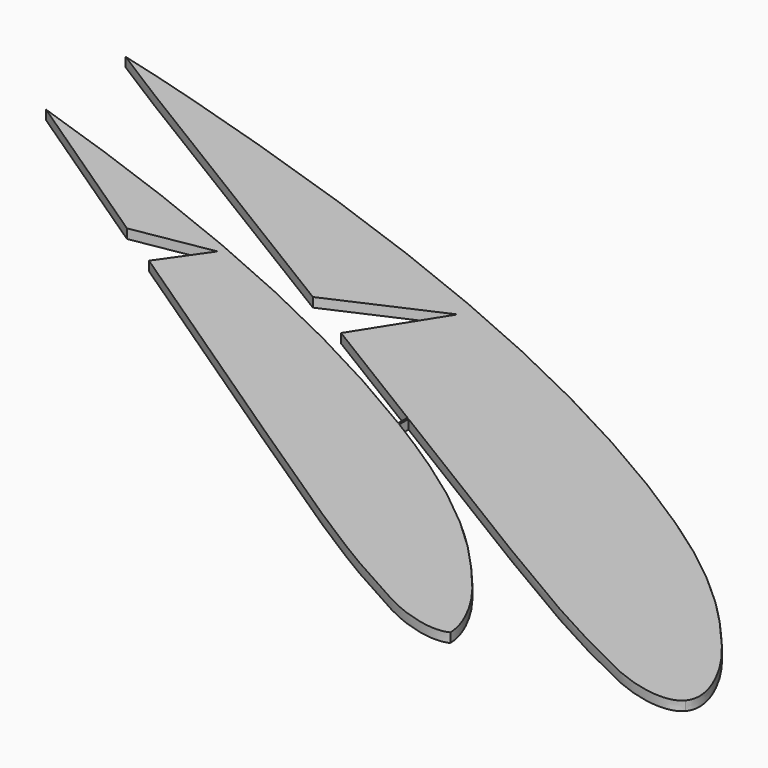
from build123d import *

# Parameters (mm, degrees)
F1_DEPTH = 2


# Not quite as in the source:
# - the dataset's text gives a spline's control points without its knots; the knots are read off the source's solid
# - a feature names something its author has since deleted; it is built from what else it names


with BuildPart() as f1:
    # F0 (on Top) → F1 (new body)
    with BuildSketch(Plane.XY):
        with BuildLine():
            add(Edge.make_bspline(
                [(34.860599786, 6.0687586182), (35.2687453157, 5.8190452704), (37.9503490475, 4.1782223052), (42.9046433804, 1.1446644855), (49.7245476866, -3.027837403), (56.54608151, -7.2008211399), (63.3647574685, -11.3765509779), (69.0485632229, -14.8494069376), (73.6045415108, -17.6232662722), (77.0228874716, -19.7002862098), (80.4388440403, -21.7712172731), (83.8571502757, -23.8323742426), (86.7081675393, -25.5302350613), (89.0084243125, -26.8828856902), (90.7408045712, -27.8935456128), (92.4769612198, -28.8998816401), (94.2144438156, -29.9024682228), (95.9476947005, -30.8994796567), (97.67369129, -31.889003941), (99.3967456723, -32.8707532075), (101.126358674, -33.8441717679), (102.8704996688, -34.8067332872), (104.6349485728, -35.7562751813), (106.4257836837, -36.6941374387), (108.2368428496, -37.6199323622), (110.0525217909, -38.5337763803), (111.8555610734, -39.4368456272), (113.6278147654, -40.3278884849), (115.3611971774, -41.2041212919), (117.0700429624, -42.0607550761), (118.7971750388, -42.8873919534), (120.2987360559, -43.539044525), (121.5536357842, -44.027474014), (122.8468885355, -44.4903446585), (124.531625858, -45.0115374905), (126.6377529307, -45.5104636967), (128.4270481511, -45.7764347039), (129.8441585723, -45.8545335174), (130.8873251545, -45.8291031583), (131.8926379099, -45.6988700343), (132.828483914, -45.43983661), (133.6579819463, -45.0271299968), (134.1089517191, -44.6391463008), (134.3025347026, -44.4182446105)],
                knots=[805.0679993481, 805.0679993481, 805.0679993481, 805.0679993481, 813.1781775179, 858.3547429355, 903.5313083532, 948.7078737709, 993.8844391885, 1039.0610046062, 1061.649287315, 1084.2375700238, 1106.8258527327, 1129.4141354415, 1152.0024181503, 1163.2965595047, 1174.5907008592, 1185.8848422136, 1197.178983568, 1208.4731249224, 1219.7672662768, 1231.0614076312, 1242.3555489857, 1253.6496903401, 1264.9438316945, 1276.2379730489, 1287.5321144033, 1298.8262557577, 1310.1203971121, 1321.4145384666, 1332.708679821, 1344.0028211754, 1355.2969625298, 1366.5911038842, 1372.2381745614, 1377.8852452386, 1389.179386593, 1400.4735279475, 1411.7676693019, 1417.4147399791, 1423.0618106563, 1428.7088813335, 1434.3559520107, 1440.0030226879, 1445.6500933651, 1445.6500933651, 1445.6500933651, 1445.6500933651], degree=3))
            add(Edge.make_bspline(
                [(134.3025347026, -44.4182446105), (134.4985490764, -44.1945684086), (134.8248159243, -43.6923009831), (135.1078544695, -42.8095001783), (135.205021821, -41.8422445125), (135.1501095293, -40.8282113605), (134.975391368, -39.7894708339), (134.7075732398, -38.7435385922), (134.3683354813, -37.7026123972), (133.841804506, -36.3291331372), (133.0760844187, -34.6508561389), (132.0561245272, -32.7309758173), (131.1567589387, -31.2285596568), (130.4187876834, -30.0885083492), (129.8574307231, -29.2631222798), (129.2885766755, -28.4642996802), (128.7105806023, -27.6857239166), (128.1224667089, -26.9217345108), (127.5240892916, -26.1675844071), (126.9126520377, -25.4155593408), (126.0792163914, -24.4101439472), (125.0044725273, -23.14313805), (123.6727030697, -21.6085195966), (122.3086179596, -20.0710503087), (120.9197072947, -18.544727339), (119.5127808585, -17.0448685527), (118.0906248287, -15.5804853344), (116.6556539097, -14.1561713196), (115.2043354173, -12.7670509391), (113.731067744, -11.4038507997), (112.2359474887, -10.06162161), (110.2113517993, -8.2930831737), (107.6229635156, -6.1178813566), (104.4430145695, -3.5839997225), (101.2076134278, -1.1457368322), (97.9237908915, 1.2091018409), (94.5952853786, 3.5053295316), (91.228268046, 5.7578295955), (86.7000179994, 8.7039617459), (82.1227805571, 11.5638270054), (77.5023902987, 14.3514293201), (74.0156610077, 16.4084086641), (70.5081197823, 18.4312591562), (66.983191083, 20.4179504986), (63.4382661844, 22.3714369923), (58.6877730154, 24.9332961185), (52.7131711017, 28.0551419964), (46.6806069198, 31.0762775575), (41.8235450338, 33.4337885791), (38.1655202683, 35.1733203209), (34.494587003, 36.8840687288), (29.5847481148, 39.1269405961), (23.4177587851, 41.8613078428), (17.2165224292, 44.5057919901), (12.2323115482, 46.572058939), (8.4826600104, 48.0979477813), (4.7239527171, 49.5999016999), (-0.2907115865, 51.5680807839), (-6.5621137407, 53.9644562837), (-12.864106821, 56.2905039474), (-17.9365378549, 58.1171933612), (-21.7532419819, 59.4699275213), (-25.5722099127, 60.8026890188), (-29.3902027457, 62.1148948136), (-33.2135123019, 63.4090298901), (-36.4095997856, 64.4746966143), (-38.972432745, 65.3199824625), (-41.537052636, 66.1599255834), (-46.0356987638, 67.6183180092), (-50.5544663128, 69.0533041025), (-54.4226479189, 70.2589031341), (-56.3562208186, 70.857081615), (-58.2915278, 71.4515221165), (-60.2400882209, 72.0459223863), (-62.1998296313, 72.639688125), (-64.1623631317, 73.2301356662), (-66.1185814879, 73.8141454773), (-68.0631750531, 74.3895135617), (-70.0051537093, 74.9580604377), (-71.9471572764, 75.5195749662), (-73.8864183513, 76.0723784332), (-76.4709863037, 76.7976496792), (-79.7065256164, 77.6826704392), (-82.3144423774, 78.3701151223), (-83.6209282279, 78.7080004811)],
                knots=[0, 0, 0, 0, 5.7179975377, 11.4359950753, 17.153992613, 22.8719901506, 28.5899876883, 34.3079852259, 40.0259827636, 45.7439803013, 57.1799753766, 68.6159704519, 80.0519655272, 85.7699630649, 91.4879606025, 97.2059581402, 102.9239556778, 108.6419532155, 114.3599507531, 120.0779482908, 125.7959458284, 137.2319409038, 148.6679359791, 160.1039310544, 171.5399261297, 182.975921205, 194.4119162803, 205.8479113556, 217.283906431, 228.7199015063, 240.1558965816, 251.5918916569, 274.4638818075, 297.3358719582, 320.2078621088, 343.0798522594, 365.95184241, 388.8238325607, 411.6958227113, 457.4398030125, 480.3117931632, 503.1837833138, 526.0557734644, 548.927763615, 571.7997537657, 594.6717439163, 640.4157242176, 686.1597045188, 709.0316946694, 731.9036848201, 754.7756749707, 777.6476651213, 823.3916454226, 869.1356257238, 892.0076158745, 914.8796060251, 937.7515961757, 960.6235863263, 1006.3675666276, 1052.1115469288, 1074.9835370795, 1097.8555272301, 1120.7275173807, 1143.5995075313, 1166.471497682, 1189.3434878326, 1200.7794829079, 1212.2154779832, 1235.0874681339, 1280.8314484351, 1292.2674435104, 1303.7034385857, 1315.139433661, 1326.5754287364, 1338.0114238117, 1349.447418887, 1360.8834139623, 1372.3194090376, 1383.7554041129, 1395.1913991882, 1406.6273942636, 1418.0633893389, 1440.9353794895, 1463.8073696401, 1463.8073696401, 1463.8073696401, 1463.8073696401], degree=3))
            add(Edge.make_bspline(
                [(-83.6209282279, 78.7080004811), (-82.4998479043, 77.9874443746), (-80.2533908905, 76.553211054), (-76.8704666528, 74.4222160876), (-73.5118161406, 72.3327832129), (-70.1615991726, 70.2687255901), (-66.7851728831, 68.2005935167), (-63.3722049541, 66.1146844339), (-59.9609837459, 64.0308472467), (-56.5489400944, 61.9470761917), (-53.7053473138, 60.2111551998), (-51.4304086553, 58.8226769605), (-49.7239011828, 57.7812203529), (-48.0184108181, 56.740398605), (-46.3394066726, 55.7156688354), (-44.6987592217, 54.7142086592), (-43.0989574675, 53.7374856774), (-41.534642881, 52.7821932861), (-39.4817271705, 51.5281794318), (-37.4489044665, 50.2859089467), (-35.3746545605, 49.0178743598), (-33.7863133878, 48.0467079366), (-32.1581010011, 47.0510308138), (-30.4900805083, 46.0309258142), (-29.0742592385, 45.1650219565), (-27.9370033118, 44.4694811815), (-26.8002344243, 43.7742386659), (-25.3791034539, 42.9050886304), (-23.1053745589, 41.5145265186), (-20.2631544361, 39.7763473135), (-16.8524824781, 37.6905803966), (-14.0102466936, 35.9524318213), (-11.7364588122, 34.5619499993), (-10.0310548349, 33.5190914776), (-8.325794231, 32.4763820972), (-6.6828148484, 31.4718315562), (-5.6098836569, 30.8158705654), (-5.108932202, 30.5096115517)],
                knots=[0, 0, 0, 0, 22.5882827088, 45.1765654177, 67.7648481265, 90.3531308353, 112.9414135441, 135.529696253, 158.1179789618, 180.7062616706, 203.2945443795, 214.5886857339, 225.8828270883, 237.1769684427, 248.4711097971, 259.7652511515, 271.059392506, 282.3535338604, 293.6476752148, 316.2359579236, 327.530099278, 338.8242406325, 350.1183819869, 361.4125233413, 372.7066646957, 378.3537353729, 384.0008060501, 395.2949474045, 406.5890887589, 429.1773714678, 451.7656541766, 474.3539368854, 485.6480782398, 496.9422195943, 508.2363609487, 519.5305023031, 529.5742922345, 529.5742922345, 529.5742922345, 529.5742922345], degree=3))
            Line((-5.108932202, 30.5096115517), (17.6389588803, 40.643003081))
            Line((17.6389588803, 40.643003081), (6.6846058821, 23.2999303896))
            add(Edge.make_bspline(
                [(6.6846058821, 23.2999303896), (6.9323313899, 23.1484621063), (7.6874850782, 22.68672343), (8.9737050889, 21.9002093392), (10.5721575546, 20.9226809598), (12.2219767669, 19.9136649735), (13.631700981, 19.0514436312), (14.7685846147, 18.3560847658), (15.9054166828, 17.6607542497), (17.3264785043, 16.7915840143), (19.6001964037, 15.4009551977), (22.4424281485, 13.6627869356), (25.853238592, 11.5772202258), (29.8421143591, 9.1383475879), (32.6938564885, 7.3943452808), (34.4085805118, 6.3453056552)],
                knots=[615.6201977517, 615.6201977517, 615.6201977517, 615.6201977517, 621.1777744928, 632.4719158472, 643.7660572017, 655.0601985561, 666.3543399105, 672.0014105877, 677.6484812649, 688.9426226193, 700.2367639737, 722.8250466826, 745.4133293914, 768.0016121002, 802.0740276243, 802.0740276243, 802.0740276243, 802.0740276243], degree=3))
            Line((34.4085805118, 6.3453056552), (34.4085805118, 8.2826344296))
            Line((34.4085805118, 8.2826344296), (34.860599786, 8.2826344296))
            Line((34.860599786, 8.2826344296), (34.860599786, 6.0687586182))
        make_face()
        with BuildLine():
            add(Edge.make_bspline(
                [(88.3839280895, -49.7027102328), (88.3835961597, -49.4131897249), (88.3426503889, -48.7793843774), (88.1724155794, -47.7849724192), (87.9013180512, -46.7388919537), (87.5587521438, -45.6980296897), (87.0277597968, -44.3248643), (86.2564798368, -42.6473266489), (85.2300320253, -40.7287109424), (84.3254995714, -39.2275787134), (83.5835584206, -38.0886631487), (83.0193032962, -37.2641780853), (82.4476216962, -36.4663018429), (81.8668488529, -35.6887169728), (81.2759916437, -34.9257608171), (80.6748904294, -34.1726825358), (80.0607239823, -33.4217691589), (79.2236253939, -32.4178865032), (78.1442438725, -31.1528832842), (76.8068305954, -29.6207778239), (75.4370647287, -28.085912989), (74.0424837191, -26.5622765557), (72.629947937, -25.0651801616), (71.2022722388, -23.6036350762), (69.7618868295, -22.1822319837), (68.305241713, -20.7961012678), (66.826703346, -19.4359776067), (65.3263540181, -18.0969070408), (63.294820031, -16.3326892644), (60.6978109426, -14.1630873664), (57.5076736263, -11.6362082054), (54.262313058, -9.2051938254), (50.9687308044, -6.8578184418), (47.6305964304, -4.5692359514), (44.2540432764, -2.3245318575), (40.0080038214, 0.4204629237), (36.8666470848, 2.3774432983), (34.860599786, 3.601533805)],
                knots=[17.8925652141, 17.8925652141, 17.8925652141, 17.8925652141, 22.8719901506, 28.5899876883, 34.3079852259, 40.0259827636, 45.7439803013, 57.1799753766, 68.6159704519, 80.0519655272, 85.7699630649, 91.4879606025, 97.2059581402, 102.9239556778, 108.6419532155, 114.3599507531, 120.0779482908, 125.7959458284, 137.2319409038, 148.6679359791, 160.1039310544, 171.5399261297, 182.975921205, 194.4119162803, 205.8479113556, 217.283906431, 228.7199015063, 240.1558965816, 251.5918916569, 274.4638818075, 297.3358719582, 320.2078621088, 343.0798522594, 365.95184241, 388.8238325607, 411.6958227113, 451.5003586634, 451.5003586634, 451.5003586634, 451.5003586634], degree=3))
            Line((34.860599786, 3.601533805), (34.860599786, 1.9013537094))
            Line((34.860599786, 1.9013537094), (34.4085805118, 1.9013537094))
            Line((34.4085805118, 1.9013537094), (34.4085805118, 3.8769267939))
            add(Edge.make_bspline(
                [(34.4085805118, 3.8769267939), (34.2597363405, 3.9674694859), (32.9567275383, 4.7588859577), (30.4910047762, 6.2367650641), (26.9952022012, 8.285426951), (23.478668504, 10.2998692035), (19.9448370857, 12.2780696838), (16.391088316, 14.2229777244), (11.6289332256, 16.7732913948), (5.6399556312, 19.880528), (-0.4067427044, 22.8867964376), (-5.2749666501, 25.2322709174), (-8.9412932745, 26.9627056092), (-12.6204561275, 28.6642939095), (-17.5411704413, 30.894874118), (-23.7215790443, 33.6137290774), (-29.9360036145, 36.2425216578), (-34.9306422078, 38.2961240955), (-38.6880554647, 39.8124600198), (-42.4544628919, 41.304813466), (-47.4792966232, 43.2601525196), (-53.7632275878, 45.6404124502), (-60.0775720534, 47.950193233), (-65.1598122116, 49.7637491863), (-68.9838338909, 51.1065819222), (-72.810063292, 52.4294177071), (-76.6352569467, 53.731682404), (-79.7234195804, 54.7669888725), (-81.5387734877, 55.3690812377), (-82.0748269579, 55.5463176388)],
                knots=[454.4888241045, 454.4888241045, 454.4888241045, 454.4888241045, 457.4398030125, 480.3117931632, 503.1837833138, 526.0557734644, 548.927763615, 571.7997537657, 594.6717439163, 640.4157242176, 686.1597045188, 709.0316946694, 731.9036848201, 754.7756749707, 777.6476651213, 823.3916454226, 869.1356257238, 892.0076158745, 914.8796060251, 937.7515961757, 960.6235863263, 1006.3675666276, 1052.1115469288, 1074.9835370795, 1097.8555272301, 1120.7275173807, 1143.5995075313, 1166.471497682, 1176.0464962651, 1176.0464962651, 1176.0464962651, 1176.0464962651], degree=3))
            add(Edge.make_bspline(
                [(-82.0748269579, 55.5463176388), (-81.6514823542, 55.2623218663), (-80.2314920702, 54.3096308948), (-78.3297225931, 53.0332109773), (-76.3095199904, 51.6768412447), (-74.762572736, 50.6380328548), (-73.1767989809, 49.5730157901), (-71.5522583041, 48.4818755603), (-70.1733443521, 47.5556767665), (-69.0657343776, 46.8117041911), (-67.9585987295, 46.0680506162), (-66.5745134384, 45.1383795229), (-64.3600543088, 43.650987153), (-61.5919203956, 41.7917676114), (-58.2701498389, 39.5607519574), (-55.5019989594, 37.701562378), (-53.2874774244, 36.214247784), (-51.6265230867, 35.0987619968), (-49.9657057672, 33.9834314558), (-48.3042303771, 32.8677401221), (-46.6450497579, 31.7536773241), (-45.4772512628, 30.9696044191), (-44.8618726805, 30.5564434009), (-44.779405515, 30.5010756906)],
                knots=[284.1357046905, 284.1357046905, 284.1357046905, 284.1357046905, 293.6476752148, 316.2359579236, 327.530099278, 338.8242406325, 350.1183819869, 361.4125233413, 372.7066646957, 378.3537353729, 384.0008060501, 395.2949474045, 406.5890887589, 429.1773714678, 451.7656541766, 474.3539368854, 485.6480782398, 496.9422195943, 508.2363609487, 519.5305023031, 530.8246436575, 542.1187850119, 543.8712452438, 543.8712452438, 543.8712452438, 543.8712452438], degree=3))
            Line((-44.779405515, 30.5010756906), (-27.7955523838, 33.4201136022))
            Line((-27.7955523838, 33.4201136022), (-34.6170857118, 23.6779543768))
            add(Edge.make_bspline(
                [(-34.6170857118, 23.6779543768), (-34.121400303, 23.3450753142), (-33.1165099045, 22.670207915), (-31.5602061291, 21.6249317798), (-29.953394086, 20.5456556935), (-28.5804202291, 19.6233990685), (-27.4731747928, 18.879624258), (-26.3659797137, 18.1358799929), (-24.9819644308, 17.2061916454), (-22.7675191381, 15.7187330401), (-19.9993731367, 13.8595239464), (-16.6774555688, 11.6287025973), (-12.248186707, 8.6544273035), (-6.712075105, 4.9359350184), (-0.0707162637, 0.4699865073), (6.5713440273, -3.9929515176), (13.2150132842, -8.4564407948), (19.8557077483, -12.9225543938), (25.3914902858, -16.6374640558), (29.8292383635, -19.6053469671), (33.1590553889, -21.8279426685), (36.4867424252, -24.0443478145), (39.8171954319, -26.2510791122), (42.5958437633, -28.0703556463), (44.8384452361, -29.5209671396), (46.5277469646, -30.6054039419), (48.2210092043, -31.6856777795), (49.9157570828, -32.7622587139), (51.6065108003, -33.8330843339), (53.2903292656, -34.8961139181), (54.9715367593, -35.9512432829), (56.6596576248, -36.9983214499), (58.3627687197, -38.0351615923), (60.086741985, -39.0598473647), (61.8375985412, -40.0739776476), (63.6091928509, -41.0769022645), (65.3859159272, -42.0680729552), (67.1504585159, -43.0479306445), (68.8847282935, -44.0144507828), (70.5807582751, -44.9645053319), (72.253086875, -45.8939160022), (73.944979232, -46.7941091817), (75.4187578859, -47.5097123622), (76.652831962, -48.0515882083), (77.9263471566, -48.5695393252), (79.5888562733, -49.1624875341), (81.6736968036, -49.7511191791), (83.4516336674, -50.093303485), (84.8653944374, -50.2317648895), (85.9096273905, -50.2507701208), (86.9204713533, -50.1633618442), (87.7466808617, -49.9721237175), (88.2137388119, -49.7849382483), (88.3839280895, -49.7027102328)],
                knots=[621.1882999755, 621.1882999755, 621.1882999755, 621.1882999755, 632.4719158472, 643.7660572017, 655.0601985561, 666.3543399105, 672.0014105877, 677.6484812649, 688.9426226193, 700.2367639737, 722.8250466826, 745.4133293914, 768.0016121002, 813.1781775179, 858.3547429355, 903.5313083532, 948.7078737709, 993.8844391885, 1039.0610046062, 1061.649287315, 1084.2375700238, 1106.8258527327, 1129.4141354415, 1152.0024181503, 1163.2965595047, 1174.5907008592, 1185.8848422136, 1197.178983568, 1208.4731249224, 1219.7672662768, 1231.0614076312, 1242.3555489857, 1253.6496903401, 1264.9438316945, 1276.2379730489, 1287.5321144033, 1298.8262557577, 1310.1203971121, 1321.4145384666, 1332.708679821, 1344.0028211754, 1355.2969625298, 1366.5911038842, 1372.2381745614, 1377.8852452386, 1389.179386593, 1400.4735279475, 1411.7676693019, 1417.4147399791, 1423.0618106563, 1428.7088813335, 1434.3559520107, 1437.8442705441, 1437.8442705441, 1437.8442705441, 1437.8442705441], degree=3))
        make_face()
        with BuildLine():
            add(Edge.make_bspline(
                [(34.4085805118, 6.3453056552), (34.5592547496, 6.2531256636), (34.7099278588, 6.1609433627), (34.860599786, 6.0687586182)],
                knots=[802.0740276243, 802.0740276243, 802.0740276243, 802.0740276243, 805.0679993481, 805.0679993481, 805.0679993481, 805.0679993481], degree=3))
            Line((34.860599786, 6.0687586182), (34.860599786, 8.2826344296))
            Line((34.860599786, 8.2826344296), (34.4085805118, 8.2826344296))
            Line((34.4085805118, 8.2826344296), (34.4085805118, 6.3453056552))
        make_face()
        with BuildLine():
            Line((34.860599786, 3.601533805), (34.860599786, 6.0687586182))
            add(Edge.make_bspline(
                [(34.4085805118, 6.3453056552), (34.5592547496, 6.2531256636), (34.7099278588, 6.1609433627), (34.860599786, 6.0687586182)],
                knots=[802.0740276243, 802.0740276243, 802.0740276243, 802.0740276243, 805.0679993481, 805.0679993481, 805.0679993481, 805.0679993481], degree=3))
            Line((34.4085805118, 6.3453056552), (34.4085805118, 3.8769267939))
            add(Edge.make_bspline(
                [(34.860599786, 3.601533805), (34.7099887343, 3.6934367022), (34.5593154632, 3.7852339304), (34.4085805118, 3.8769267939)],
                knots=[451.5003586634, 451.5003586634, 451.5003586634, 451.5003586634, 454.4888241045, 454.4888241045, 454.4888241045, 454.4888241045], degree=3))
        make_face()
        with BuildLine():
            Line((34.860599786, 1.9013537094), (34.860599786, 3.601533805))
            add(Edge.make_bspline(
                [(34.860599786, 3.601533805), (34.7099887343, 3.6934367022), (34.5593154632, 3.7852339304), (34.4085805118, 3.8769267939)],
                knots=[451.5003586634, 451.5003586634, 451.5003586634, 451.5003586634, 454.4888241045, 454.4888241045, 454.4888241045, 454.4888241045], degree=3))
            Line((34.4085805118, 3.8769267939), (34.4085805118, 1.9013537094))
            Line((34.4085805118, 1.9013537094), (34.860599786, 1.9013537094))
        make_face()
    extrude(amount=F1_DEPTH)


solid = f1.part
